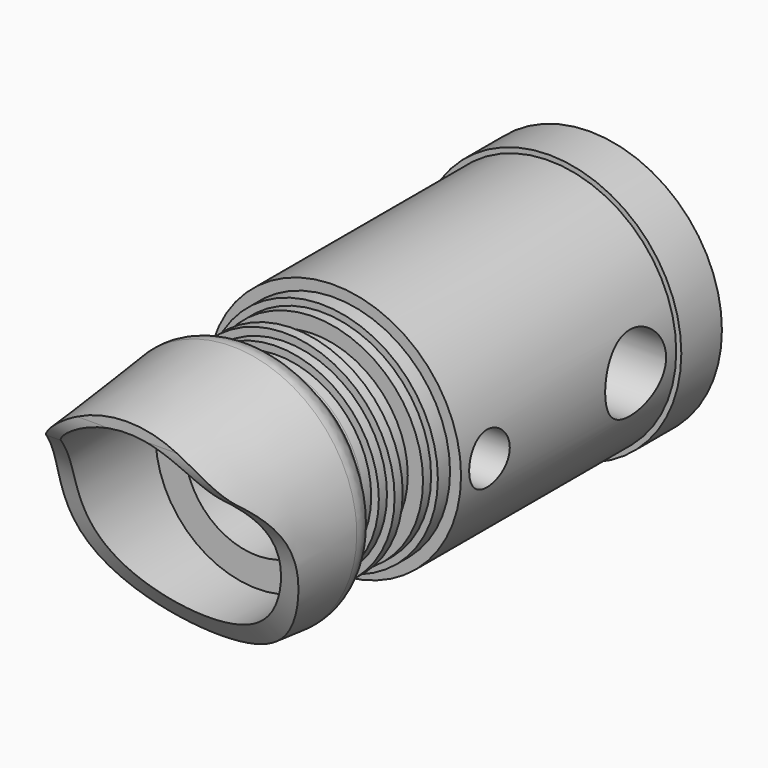
from build123d import *

# Parameters (mm, degrees)
F0_R         = 25
F1_DEPTH     = 53
F2_R         = 26
F3_DEPTH     = 10
F4_R         = 22.8291590373
F5_DEPTH     = 3
F6_R         = 21.5
F7_DEPTH     = 2
F8_R         = 18.5
F9_DEPTH     = 5
F10_R        = 21.5
F11_DEPTH    = 2
F12_R        = 20
F13_DEPTH    = 2
F14_R        = 18.5
F15_DEPTH    = 2
F16_R        = 25
F17_DEPTH    = 35
F18_R        = 20
F19_DEPTH    = 32
F20_S5_R     = 18.5
F20_T6_DEPTH = 37
F22_R        = 5
F25_DEPTH    = 52.3
F26_T1_DEPTH = 27.7214737536
F26_T3_DEPTH = 27.7214737536
F27_R        = 14.25
F28_DEPTH    = 128
F29_R        = 5
F30_DEPTH    = 39.2


# Not quite as in the source:
# - a fillet or chamfer that OpenCascade refuses, or shapes differently, is made with other operations: its cross-section is extruded or revolved along the edge and cut away or added


with BuildPart() as f1:
    # F0 (on Front) → F1 (new body)
    with BuildSketch(Plane.XZ):
        Circle(F0_R)
    extrude(amount=F1_DEPTH)

    # F2 (on face) → F3 (join)
    with BuildSketch(Plane(origin=(0, 0, 0), x_dir=(-1, 0, 0), z_dir=(0, 1, 0))):
        Circle(F2_R)
    extrude(amount=F3_DEPTH)

    # F4 (on face) → F5 (join)
    with BuildSketch(Plane.XZ.offset(53)):
        Circle(F4_R)
    extrude(amount=F5_DEPTH)

    # F6 (on face) → F7 (join)
    with BuildSketch(Plane.XZ.offset(56)):
        Circle(F6_R)
    extrude(amount=F7_DEPTH)

    # F8 (on face) → F9 (join)
    with BuildSketch(Plane.XZ.offset(58)):
        Circle(F8_R)
    extrude(amount=F9_DEPTH)

    # F10 (on face) → F11 (join)
    with BuildSketch(Plane.XZ.offset(63)):
        Circle(F10_R)
    extrude(amount=F11_DEPTH)

    # F12 (on face) → F13 (join)
    with BuildSketch(Plane.XZ.offset(65)):
        Circle(F12_R)
    extrude(amount=F13_DEPTH)

    # F14 (on face) → F15 (join)
    with BuildSketch(Plane.XZ.offset(67)):
        Circle(F14_R)
    extrude(amount=F15_DEPTH)

    # F16 (on face) → F17 (join)
    with BuildSketch(Plane.XZ.offset(69)):
        Circle(F16_R)
    extrude(amount=F17_DEPTH)

    # F18 (on face) → F19 (cut)
    with BuildSketch(Plane.XZ.offset(104)):
        Circle(F18_R)
    extrude(amount=-F19_DEPTH, mode=Mode.SUBTRACT)

    # F20: chamfer of 7 on 1 edges, made by hand


with BuildPart() as f20_tool2:
    # F20_s3 → F20_t4 (revolve)
    with BuildSketch(Plane.XY):
        Polygon((25, -76), (18, -69), (25, -69), align=None)
    revolve(axis=Axis((0, -69, 0), (0, -1, 0)))

    # F20_s5 → F20_t6 (cut, symmetric)
    with BuildSketch(Plane.XZ.offset(72.5)):
        Circle(F20_S5_R)
    extrude(amount=F20_T6_DEPTH, both=True, mode=Mode.SUBTRACT)


with BuildPart() as f1_1:
    add(f1.part)

    # F20_t1: cut F20_tool2
    add(f20_tool2.part, mode=Mode.SUBTRACT)

    # F21: chamfer of 3 x 30 on 1 edges, made by hand

    # F21_s1 → F21_t2 (revolve, cut)
    with BuildSketch(Plane.XY):
        Polygon((25, -74), (22, -104), (25, -104), align=None)
    revolve(axis=Axis((0, -104, 0), (0, -1, 0)), mode=Mode.SUBTRACT)

    # F22
    f22_edges = [f1_1.edges().sort_by_distance(p)[0] for p in [
        (-24.818182, -75.818182, 0),
    ]]
    fillet(f22_edges, radius=F22_R)

    # F24 (on offset) → F25 (cut)
    with BuildSketch(Plane.YZ.offset(26.9)):
        with BuildLine():
            Line((-78, -31.0485586524), (-78, -28.3997934312))
            add(Edge.make_bspline(
                [(-78, -28.3997934312), (-98.6184179783, -3.1667915173), (-82.4469923973, 1.2942913454), (-107.4011772871, 17.0474909246)],
                knots=[0, 0, 0, 0, 54.1284110351, 54.1284110351, 54.1284110351, 54.1284110351], degree=3))
            Line((-107.4011772871, 17.0474909246), (-107.4011772871, -31.0485586524))
            Line((-107.4011772871, -31.0485586524), (-78, -31.0485586524))
        make_face()
    extrude(amount=-F25_DEPTH, mode=Mode.SUBTRACT)

    # F26: fillet of radius 10 on 2 edges, made by hand

    # F26_s2 → F26_t1 (cut)
    with BuildSketch(Plane.YZ.offset(1.0087475172)):
        with BuildLine():
            ThreePointArc((-100.3409030979, 12.0407262021), (-103.0393566379, 15.4967106846), (-104.0004, 19.7747798644))
            Line((-104.0004, 19.7747798644), (-105.00064, 19.7747798644))
            ThreePointArc((-105.00064, 19.7747798644), (-105.00024, 17.2850901727), (-105.00024, 14.795400481))
            Line((-105.00024, 14.795400481), (-104.5724569812, 13.9751730356))
            ThreePointArc((-104.5724569812, 13.9751730356), (-102.7441847483, 12.6535319788), (-100.9751934077, 11.2673208359))
            Line((-100.9751934077, 11.2673208359), (-100.3409030979, 12.0407262021))
        make_face()
    extrude(amount=F26_T1_DEPTH, mode=Mode.SUBTRACT)

    # F26_s4 → F26_t3 (cut)
    with BuildSketch(Plane.YZ.offset(-28.7302212708)):
        with BuildLine():
            ThreePointArc((-100.3409030979, 12.0407262021), (-103.0393566379, 15.4967106846), (-104.0004, 19.7747798644))
            Line((-104.0004, 19.7747798644), (-105.00064, 19.7747798644))
            ThreePointArc((-105.00064, 19.7747798644), (-105.00024, 17.2850901727), (-105.00024, 14.795400481))
            Line((-105.00024, 14.795400481), (-104.5724569812, 13.9751730356))
            ThreePointArc((-104.5724569812, 13.9751730356), (-102.7441847483, 12.6535319788), (-100.9751934077, 11.2673208359))
            Line((-100.9751934077, 11.2673208359), (-100.3409030979, 12.0407262021))
        make_face()
    extrude(amount=F26_T3_DEPTH, mode=Mode.SUBTRACT)

    # F27 (on face) → F28 (cut)
    with BuildSketch(Plane(origin=(0, 10, 0), x_dir=(-1, 0, 0), z_dir=(0, 1, 0))):
        Circle(F27_R)
    extrude(amount=-F28_DEPTH, mode=Mode.SUBTRACT)

    # F29 (on Right) → F30 (cut)
    with BuildSketch(Plane.YZ):
        with BuildLine():
            ThreePointArc((-17.5, 0), (-10, -7.5), (-2.5, 0))
            Line((-2.5, 0), (-10, 0))
            Line((-10, 0), (-17.5, 0))
        make_face()
        with BuildLine():
            Line((-10, 0), (-2.5, 0))
            ThreePointArc((-2.5, 0), (-10, 7.5), (-17.5, 0))
            Line((-17.5, 0), (-10, 0))
        make_face()
        with Locations((-46, 0)):
            Circle(F29_R)
    extrude(amount=F30_DEPTH, mode=Mode.SUBTRACT)


solid = f1_1.part
